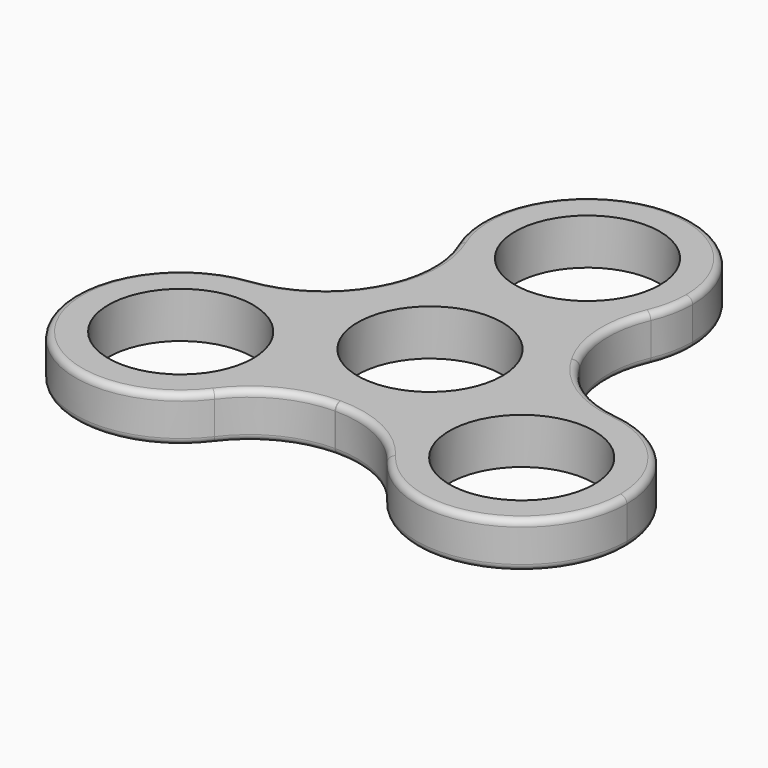
from build123d import *

# Parameters (mm, degrees)
F0_R     = 11.025
F1_DEPTH = 7
F2_R     = 1


with BuildPart() as f1:
    # F0 (on Top) → F1 (new body)
    with BuildSketch(Plane.XY):
        with BuildLine():
            ThreePointArc((14.7181475974, 23.6614862702), (15.6948867509, 26.7640836111), (16.025, 30))
            ThreePointArc((16.025, 30), (-3.2359163889, 45.6948867509), (-14.7181475974, 23.6614862702))
            ThreePointArc((-14.7181475974, 23.6614862702), (-11.9828737003, 19.359917158), (-8.0350731173, 16.135))
            ThreePointArc((-8.0350731173, 16.135), (0, 18.025), (8.0350731173, 16.135))
            ThreePointArc((8.0350731173, 16.135), (11.9828737003, 19.359917158), (14.7181475974, 23.6614862702))
        make_face()
        with Locations((0, 30)):
            Circle(F0_R, mode=Mode.SUBTRACT)
        with BuildLine():
            ThreePointArc((-8.0350731173, 16.135), (-11.9828737003, 19.359917158), (-14.7181475974, 23.6614862702))
            ThreePointArc((-14.7181475974, 23.6614862702), (-13.4190857224, 16.250871043), (-15.58998593, 9.0472627741))
            ThreePointArc((-15.58998593, 9.0472627741), (-12.3326744258, 13.1455607149), (-8.0350731173, 16.135))
        make_face()
        with BuildLine():
            ThreePointArc((15.58998593, 9.0472627741), (13.4190857224, 16.250871043), (14.7181475974, 23.6614862702))
            ThreePointArc((14.7181475974, 23.6614862702), (11.9828737003, 19.359917158), (8.0350731173, 16.135))
            ThreePointArc((8.0350731173, 16.135), (12.3326744258, 13.1455607149), (15.58998593, 9.0472627741))
        make_face()
        with BuildLine():
            ThreePointArc((8.0350731173, 16.135), (0, 13.975), (-8.0350731173, 16.135))
            ThreePointArc((-8.0350731173, 16.135), (-12.3326744258, 13.1455607149), (-15.58998593, 9.0472627741))
            ThreePointArc((-15.58998593, 9.0472627741), (-15.6101079032, 9.0125), (-15.6301523621, 8.9776924729))
            ThreePointArc((-15.6301523621, 8.9776924729), (-17.5507267389, 4.1076289919), (-17.9908564487, -1.1089225592))
            ThreePointArc((-17.9908564487, -1.1089225592), (-12.1092289741, -6.9762107854), (-9.9557621135, -15))
            ThreePointArc((-9.9557621135, -15), (-9.955767418, -15.0130387247), (-9.9557833314, -15.0260774408))
            ThreePointArc((-9.9557833314, -15.0260774408), (-5.2180523132, -17.2531897067), (-0.0401664321, -18.024955247))
            ThreePointArc((-0.0401664321, -18.024955247), (0, -18.025), (0.0401664321, -18.024955247))
            ThreePointArc((0.0401664321, -18.024955247), (5.2180523132, -17.2531897067), (9.9557833314, -15.0260774408))
            ThreePointArc((9.9557833314, -15.0260774408), (12.1027050179, -6.9875), (17.9908564487, -1.1089225592))
            ThreePointArc((17.9908564487, -1.1089225592), (18.0164620901, -0.554724036), (18.025, 0))
            ThreePointArc((18.025, 0), (17.4160001339, 4.6458114831), (15.6301523621, 8.9776924729))
            ThreePointArc((15.6301523621, 8.9776924729), (15.6101079032, 9.0125), (15.58998593, 9.0472627741))
            ThreePointArc((15.58998593, 9.0472627741), (12.3326744258, 13.1455607149), (8.0350731173, 16.135))
        make_face()
        Circle(F0_R, mode=Mode.SUBTRACT)
        with BuildLine():
            ThreePointArc((-17.9908564487, -1.1089225592), (-17.5507267389, 4.1076289919), (-15.6301523621, 8.9776924729))
            ThreePointArc((-15.6301523621, 8.9776924729), (-20.783210018, 3.4958336097), (-27.850522, 0.9155465808))
            ThreePointArc((-27.850522, 0.9155465808), (-22.7576169242, 0.6975144557), (-17.9908564487, -1.1089225592))
        make_face()
        with BuildLine():
            ThreePointArc((27.850522, 0.9155465808), (20.783210018, 3.4958336097), (15.6301523621, 8.9776924729))
            ThreePointArc((15.6301523621, 8.9776924729), (17.4160001339, 4.6458114831), (18.025, 0))
            ThreePointArc((18.025, 0), (18.0164620901, -0.554724036), (17.9908564487, -1.1089225592))
            ThreePointArc((17.9908564487, -1.1089225592), (22.7576169242, 0.6975144557), (27.850522, 0.9155465808))
        make_face()
        with BuildLine():
            ThreePointArc((-9.9557833314, -15.0260774408), (-15.6101079032, -9.0125), (-17.9908564487, -1.1089225592))
            ThreePointArc((-17.9908564487, -1.1089225592), (-22.7576169242, 0.6975144557), (-27.850522, 0.9155465808))
            ThreePointArc((-27.850522, 0.9155465808), (-39.8588192092, -23.0125), (-13.1323744027, -24.5770328511))
            ThreePointArc((-13.1323744027, -24.5770328511), (-10.7747432239, -20.0574316138), (-9.9557833314, -15.0260774408))
        make_face()
        with Locations((-25.9807621135, -15)):
            Circle(F0_R, mode=Mode.SUBTRACT)
        with BuildLine():
            ThreePointArc((42.0057621135, -15), (37.9549745549, -4.3501708272), (27.850522, 0.9155465808))
            ThreePointArc((27.850522, 0.9155465808), (22.7576169242, 0.6975144557), (17.9908564487, -1.1089225592))
            ThreePointArc((17.9908564487, -1.1089225592), (15.6101079032, -9.0125), (9.9557833314, -15.0260774408))
            ThreePointArc((9.9557833314, -15.0260774408), (10.7747432239, -20.0574316138), (13.1323744027, -24.5770328511))
            ThreePointArc((13.1323744027, -24.5770328511), (31.0258196917, -30.2101288303), (42.0057621135, -15))
        make_face()
        with Locations((25.9807621135, -15)):
            Circle(F0_R, mode=Mode.SUBTRACT)
        with BuildLine():
            ThreePointArc((-0.0401664321, -18.024955247), (-5.2180523132, -17.2531897067), (-9.9557833314, -15.0260774408))
            ThreePointArc((-9.9557833314, -15.0260774408), (-10.7747432239, -20.0574316138), (-13.1323744027, -24.5770328511))
            ThreePointArc((-13.1323744027, -24.5770328511), (-7.3641242956, -19.7467046526), (-0.0401664321, -18.024955247))
        make_face()
        with BuildLine():
            ThreePointArc((13.1323744027, -24.5770328511), (10.7747432239, -20.0574316138), (9.9557833314, -15.0260774408))
            ThreePointArc((9.9557833314, -15.0260774408), (5.2180523132, -17.2531897067), (0.0401664321, -18.024955247))
            ThreePointArc((0.0401664321, -18.024955247), (7.3641242956, -19.7467046526), (13.1323744027, -24.5770328511))
        make_face()
        with BuildLine():
            ThreePointArc((-9.9557621135, -15), (-12.1092289741, -6.9762107854), (-17.9908564487, -1.1089225592))
            ThreePointArc((-17.9908564487, -1.1089225592), (-15.6101079032, -9.0125), (-9.9557833314, -15.0260774408))
            ThreePointArc((-9.9557833314, -15.0260774408), (-9.955767418, -15.0130387247), (-9.9557621135, -15))
        make_face()
        with BuildLine():
            ThreePointArc((8.0350731173, 16.135), (0, 18.025), (-8.0350731173, 16.135))
            ThreePointArc((-8.0350731173, 16.135), (0, 13.975), (8.0350731173, 16.135))
        make_face()
        with BuildLine():
            ThreePointArc((9.9557833314, -15.0260774408), (15.6101079032, -9.0125), (17.9908564487, -1.1089225592))
            ThreePointArc((17.9908564487, -1.1089225592), (12.1027050179, -6.9875), (9.9557833314, -15.0260774408))
        make_face()
    extrude(amount=F1_DEPTH)

    # F2
    f2_edges = [f1.edges().sort_by_distance(p)[0] for p in [
        (14.718148, 23.661486, 3.5),
        (-14.718148, 23.661486, 3.5),
        (0, 46.025, 0),
        (0, 46.025, 7),
        (-15.589986, 9.047263, 3.5),
        (-13.419086, 16.250871, 0),
        (-13.419086, 16.250871, 7),
        (-15.630152, 8.977692, 3.5),
        (-27.850522, 0.915547, 3.5),
        (-20.78321, 3.495834, 0),
        (-20.78321, 3.495834, 7),
        (-13.132374, -24.577033, 3.5),
        (-39.858819, -23.0125, 0),
        (-39.858819, -23.0125, 7),
        (0.040166, -18.024955, 3.5),
        (13.132374, -24.577033, 3.5),
        (7.364124, -19.746705, 0),
        (7.364124, -19.746705, 7),
    ]]
    fillet(f2_edges, radius=F2_R)


solid = f1.part
